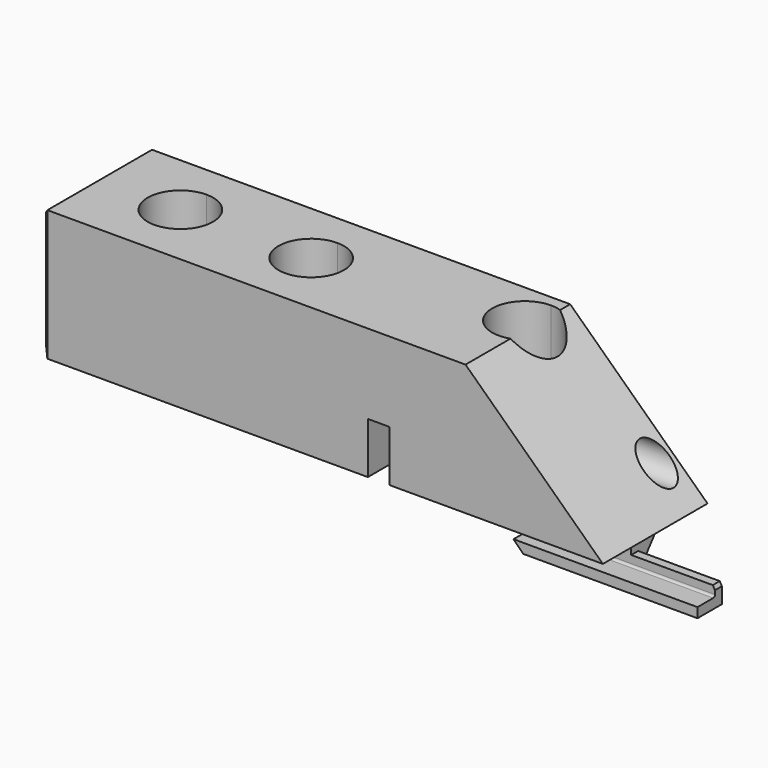
from build123d import *

# Parameters (mm, degrees)
F0_W         = 29.62
F0_H         = 7.2
F1_DEPTH     = 6
F3_DEPTH     = 6
F5_DEPTH     = 6
F6_W         = 1
F6_H         = 6
F7_DEPTH     = 2.35
F8_W         = 3.025
F8_H         = 1.2
F9_DEPTH     = 9.191
F11_DEPTH    = 9.191
F12_W        = 0.625
F12_H        = 0.45
F13_DEPTH    = 9.191
F14_R        = 0.1
F16_DEPTH    = 3.84
F18_DEPTH    = 0.4
F20_DEPTH    = 6
F21_R        = 2.5
F22_DEPTH    = 3
F24_DEPTH    = 29.621
F25_T1_DEPTH = 7.5430097928
F25_T3_DEPTH = 7.5430097928
F27_DEPTH    = 6


# Not quite as in the source:
# - a fillet or chamfer that OpenCascade refuses, or shapes differently, is made with other operations: its cross-section is extruded or revolved along the edge and cut away or added


with BuildPart() as f1:
    # F0 (on Front) → F1 (new body)
    with BuildSketch(Plane.XZ):
        Rectangle(F0_W, F0_H)
    extrude(amount=-F1_DEPTH)

    # F2 (on face) → F3 (cut, through all)
    with BuildSketch(Plane.XZ):
        Polygon((10.97, -2.4), (14.81, -2.4), (14.81, 3.6), (4.67, 3.6), align=None)
    extrude(amount=-F3_DEPTH, mode=Mode.SUBTRACT)

    # F4 (on face) → F5 (cut, through all)
    with BuildSketch(Plane.XZ):
        Polygon((6.82, -3.6), (5.62, -2.4), (-14.81, -2.4), (-14.81, -3.6), align=None)
    extrude(amount=-F5_DEPTH, mode=Mode.SUBTRACT)

    # F6 (on face) → F7 (cut)
    with BuildSketch(Plane(origin=(0, 0, -2.4), x_dir=(1, 0, 0), z_dir=(0, 0, -1))):
        with Locations((0.69, -3)):
            Rectangle(F6_W, F6_H)
    extrude(amount=-F7_DEPTH, mode=Mode.SUBTRACT)

    # F8 (on face) → F9 (cut, through all)
    with BuildSketch(Plane.YZ.offset(14.81)):
        with Locations((4.4875, -3)):
            Rectangle(F8_W, F8_H)
    extrude(amount=-F9_DEPTH, mode=Mode.SUBTRACT)

    # F10 (on face) → F11 (cut, through all)
    with BuildSketch(Plane.YZ.offset(14.81)):
        Polygon((2.025, -3.6), (2.975, -3.6), (2.975, -2.4), align=None)
    extrude(amount=-F11_DEPTH, mode=Mode.SUBTRACT)

    # F12 (on face) → F13 (cut, through all)
    with BuildSketch(Plane.YZ.offset(14.81)):
        with Locations((0.3125, -3.375)):
            Rectangle(F12_W, F12_H)
        Polygon((0, -3.15), (0.625, -3.15), (1.625, -3.15), (1.625, -2.4), (0, -2.4), align=None)
    extrude(amount=-F13_DEPTH, mode=Mode.SUBTRACT)

    # F14
    f14_edges = [f1.edges().sort_by_distance(p)[0] for p in [
        (10.59, 1.625, -3.15),
    ]]
    fillet(f14_edges, radius=F14_R)

    # F15 (on face) → F16 (cut)
    with BuildSketch(Plane.YZ.offset(14.81)):
        Polygon((2.025, -2.7), (2.025, -3.6), (2.975, -2.4), (1.625, -2.4), (1.625, -2.7), align=None)
    extrude(amount=-F16_DEPTH, mode=Mode.SUBTRACT)

    # F17 (on face) → F18 (cut, through all)
    with BuildSketch(Plane.XZ.offset(-1.625)):
        Polygon((14.81, -2.8732050808), (14.81, -2.7), (14.71, -2.7), align=None)
    extrude(amount=-F18_DEPTH, mode=Mode.SUBTRACT)

    # F19 (on face) → F20 (cut, through all)
    with BuildSketch(Plane(origin=(0, 0, -2.4), x_dir=(1, 0, 0), z_dir=(0, 0, -1))):
        with BuildLine():
            ThreePointArc((-3.31, -3), (-5.8706601718, -1.9393398282), (-4.81, -4.5))
            ThreePointArc((-4.81, -4.5), (-3.7493398282, -4.0606601718), (-3.31, -3))
        make_face()
        with BuildLine():
            ThreePointArc((-9.31, -3), (-11.8706601718, -1.9393398282), (-10.81, -4.5))
            ThreePointArc((-10.81, -4.5), (-9.7493398282, -4.0606601718), (-9.31, -3))
        make_face()
    extrude(amount=-F20_DEPTH, mode=Mode.SUBTRACT)

    # F21 (on face) → F22 (cut)
    with BuildSketch(Plane(origin=(0, 0, -2.4), x_dir=(1, 0, 0), z_dir=(0, 0, -1))):
        with Locations((-10.81, -3)):
            Circle(F21_R)
        with Locations((-4.81, -3)):
            Circle(F21_R)
    extrude(amount=-F22_DEPTH, mode=Mode.SUBTRACT)

    # F23 (on face) → F24 (cut, through all)
    with BuildSketch(Plane(origin=(-14.81, 0, 0), x_dir=(0, -1, 0), z_dir=(-1, 0, 0))):
        with BuildLine():
            ThreePointArc((-5.79, -0.9), (-5.05, -1.64), (-4.31, -0.9))
            ThreePointArc((-4.31, -0.9), (-5.05, -0.16), (-5.79, -0.9))
        make_face()
    extrude(amount=-F24_DEPTH, mode=Mode.SUBTRACT)

    # F25: chamfer of 0.3 on 4 edges, made by hand

    # F25_s2 → F25_t1 (cut)
    with BuildSketch(Plane.XY.offset(-3.1715048964)):
        Polygon((-14.51, 0), (-14.81, 0.3), (-14.81, 0), align=None)
        Polygon((-14.51, 6), (-14.81, 5.7), (-14.81, 6), align=None)
    extrude(amount=F25_T1_DEPTH, mode=Mode.SUBTRACT)

    # F25_s4 → F25_t3 (cut)
    with BuildSketch(Plane.XZ.offset(-6.7715048964)):
        Polygon((-14.51, 3.6), (-14.81, 3.3), (-14.81, 3.6), align=None)
        Polygon((-14.81, -2.1), (-14.51, -2.4), (-14.81, -2.4), align=None)
    extrude(amount=F25_T3_DEPTH, mode=Mode.SUBTRACT)

    # F26 (on face) → F27 (cut, through all)
    with BuildSketch(Plane(origin=(0, 0, -2.4), x_dir=(1, 0, 0), z_dir=(0, 0, -1))):
        with BuildLine():
            ThreePointArc((4.19, -5.5), (5.2506601718, -5.0606601718), (5.69, -4))
            ThreePointArc((5.69, -4), (3.1293398282, -2.9393398282), (4.19, -5.5))
        make_face()
    extrude(amount=-F27_DEPTH, mode=Mode.SUBTRACT)


solid = f1.part
